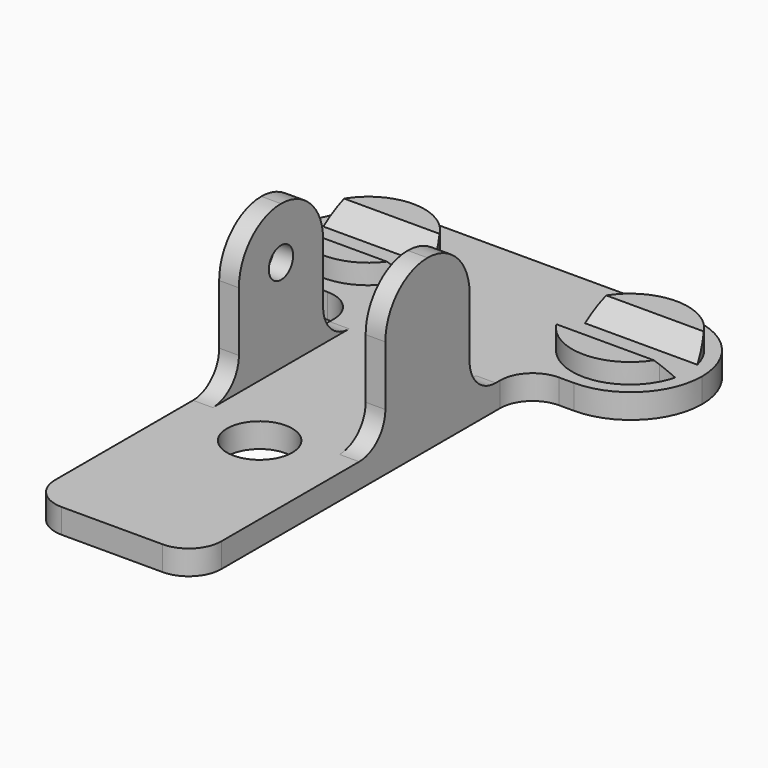
from build123d import *

# Parameters (mm, degrees)
F0_R       = 5
F1_DEPTH   = 3.75
F0_W       = 3.02
F0_H       = 16.12
F2_DEPTH   = 25.93
F3_DEPTH   = 6.79
F4_DEPTH   = 6.79
F5_SIZE2   = 3.03999
F5_SIZE    = 2.64999
F5_2_SIZE2 = 3.03999
F5_2_SIZE  = 2.64999
F6_SIZE2   = 2.64999
F6_SIZE    = 3.03999
F6_2_SIZE2 = 2.64999
F6_2_SIZE  = 3.03999
F7_R       = 2.33
F8_DEPTH   = 25
F9_R       = 8.05999
F10_R      = 5
F11_R      = 10.89999


# Not quite as in the source:
# - a fillet or chamfer is up to 0.001 mm smaller than in the source, because OpenCascade refuses the exact size


with BuildPart() as f1:
    # F0 (on Top) → F1 (new body)
    with BuildSketch(Plane.XY):
        Polygon((-30.935, 0), (-12.725, 0), (12.725, 0), (30.935, 0), (30.935, 21.8), (-30.935, 21.8), align=None)
        with BuildLine():
            ThreePointArc((-11.9316907323, 12.91), (-11.7843146524, 12.0027843216), (-11.735, 11.085))
            ThreePointArc((-11.735, 11.085), (-11.8230688054, 9.8599030561), (-12.0854641032, 8.66))
            ThreePointArc((-12.0854641032, 8.66), (-12.4738263465, 7.6050242897), (-12.9970143092, 6.61))
            ThreePointArc((-12.9970143092, 6.61), (-20.3, 2.52), (-27.6029856908, 6.61))
            ThreePointArc((-27.6029856908, 6.61), (-28.1261736535, 7.6050242897), (-28.5145358968, 8.66))
            ThreePointArc((-28.5145358968, 8.66), (-28.8593991283, 10.7753040808), (-28.6683092677, 12.91))
            ThreePointArc((-28.6683092677, 12.91), (-28.2468859573, 14.2797188579), (-27.6029856908, 15.56))
            ThreePointArc((-27.6029856908, 15.56), (-20.3, 19.65), (-12.9970143092, 15.56))
            ThreePointArc((-12.9970143092, 15.56), (-12.3531140427, 14.2797188579), (-11.9316907323, 12.91))
        make_face(mode=Mode.SUBTRACT)
        with BuildLine():
            ThreePointArc((28.6065440218, 12.91), (28.8001487986, 11.8553299132), (28.865, 10.785))
            ThreePointArc((28.865, 10.785), (28.8001487986, 9.7146700868), (28.6065440218, 8.66))
            ThreePointArc((28.6065440218, 8.66), (28.2771488358, 7.6105658536), (27.8203324738, 6.61))
            ThreePointArc((27.8203324738, 6.61), (20, 1.92), (12.1796675262, 6.61))
            ThreePointArc((12.1796675262, 6.61), (11.7228511642, 7.6105658536), (11.3934559782, 8.66))
            ThreePointArc((11.3934559782, 8.66), (11.135, 10.785), (11.3934559782, 12.91))
            ThreePointArc((11.3934559782, 12.91), (11.8536949602, 14.2815610531), (12.5308902806, 15.56))
            ThreePointArc((12.5308902806, 15.56), (20, 19.65), (27.4691097194, 15.56))
            ThreePointArc((27.4691097194, 15.56), (28.1463050398, 14.2815610531), (28.6065440218, 12.91))
        make_face(mode=Mode.SUBTRACT)
        Polygon((12.725, 0), (-12.725, 0), (-12.725, -10.84), (-9.705, -10.84), (-9.705, -26.96), (-12.725, -26.96), (-12.725, -63.35), (12.725, -63.35), (12.725, -26.96), (9.705, -26.96), (9.705, -10.84), (12.725, -10.84), align=None)
        with Locations((0, -35.12)):
            Circle(F0_R, mode=Mode.SUBTRACT)
        with BuildLine():
            ThreePointArc((-12.0854641032, 8.66), (-11.8230688054, 9.8599030561), (-11.735, 11.085))
            ThreePointArc((-11.735, 11.085), (-11.7843146524, 12.0027843216), (-11.9316907323, 12.91))
            Line((-11.9316907323, 12.91), (-28.6683092677, 12.91))
            ThreePointArc((-28.6683092677, 12.91), (-28.8593991283, 10.7753040808), (-28.5145358968, 8.66))
            Line((-28.5145358968, 8.66), (-12.0854641032, 8.66))
        make_face()
        with BuildLine():
            ThreePointArc((28.6065440218, 8.66), (28.8001487986, 9.7146700868), (28.865, 10.785))
            ThreePointArc((28.865, 10.785), (28.8001487986, 11.8553299132), (28.6065440218, 12.91))
            Line((28.6065440218, 12.91), (11.3934559782, 12.91))
            ThreePointArc((11.3934559782, 12.91), (11.135, 10.785), (11.3934559782, 8.66))
            Line((11.3934559782, 8.66), (28.6065440218, 8.66))
        make_face()
    extrude(amount=F1_DEPTH)

    # F0 (on Top) → F2 (join)
    with BuildSketch(Plane.XY):
        with Locations((-11.215, -18.9)):
            Rectangle(F0_W, F0_H)
        with Locations((11.215, -18.9)):
            Rectangle(F0_W, F0_H)
    extrude(amount=F2_DEPTH)

    # F0 (on Top) → F3 (join)
    with BuildSketch(Plane.XY):
        with BuildLine():
            Line((-27.6029856908, 15.56), (-12.9970143092, 15.56))
            ThreePointArc((-12.9970143092, 15.56), (-20.3, 19.65), (-27.6029856908, 15.56))
        make_face()
        with BuildLine():
            ThreePointArc((-27.6029856908, 6.61), (-20.3, 2.52), (-12.9970143092, 6.61))
            Line((-12.9970143092, 6.61), (-27.6029856908, 6.61))
        make_face()
        with BuildLine():
            ThreePointArc((12.1796675262, 6.61), (20, 1.92), (27.8203324738, 6.61))
            Line((27.8203324738, 6.61), (12.1796675262, 6.61))
        make_face()
        with BuildLine():
            Line((12.5308902806, 15.56), (27.4691097194, 15.56))
            ThreePointArc((27.4691097194, 15.56), (20, 19.65), (12.5308902806, 15.56))
        make_face()
    extrude(amount=F3_DEPTH)

    # F0 (on Top) → F4 (join)
    with BuildSketch(Plane.XY):
        with BuildLine():
            Line((-28.6683092677, 12.91), (-11.9316907323, 12.91))
            ThreePointArc((-11.9316907323, 12.91), (-12.3531140427, 14.2797188579), (-12.9970143092, 15.56))
            Line((-12.9970143092, 15.56), (-27.6029856908, 15.56))
            ThreePointArc((-27.6029856908, 15.56), (-28.2468859573, 14.2797188579), (-28.6683092677, 12.91))
        make_face()
        with BuildLine():
            ThreePointArc((-12.9970143092, 6.61), (-12.4738263465, 7.6050242897), (-12.0854641032, 8.66))
            Line((-12.0854641032, 8.66), (-28.5145358968, 8.66))
            ThreePointArc((-28.5145358968, 8.66), (-28.1261736535, 7.6050242897), (-27.6029856908, 6.61))
            Line((-27.6029856908, 6.61), (-12.9970143092, 6.61))
        make_face()
        with BuildLine():
            ThreePointArc((27.8203324738, 6.61), (28.2771488358, 7.6105658536), (28.6065440218, 8.66))
            Line((28.6065440218, 8.66), (11.3934559782, 8.66))
            ThreePointArc((11.3934559782, 8.66), (11.7228511642, 7.6105658536), (12.1796675262, 6.61))
            Line((12.1796675262, 6.61), (27.8203324738, 6.61))
        make_face()
        with BuildLine():
            Line((11.3934559782, 12.91), (28.6065440218, 12.91))
            ThreePointArc((28.6065440218, 12.91), (28.1463050398, 14.2815610531), (27.4691097194, 15.56))
            Line((27.4691097194, 15.56), (12.5308902806, 15.56))
            ThreePointArc((12.5308902806, 15.56), (11.8536949602, 14.2815610531), (11.3934559782, 12.91))
        make_face()
    extrude(amount=F4_DEPTH)

    # F5 (size 2.65 and 3.04 in the source; OpenCascade refuses exactly that, so slightly less here)
    f5_edges = [f1.edges().sort_by_distance(p)[0] for p in [
        (-20.3, 12.91, 6.79),
    ]]
    f5_side = f1.faces().sort_by_distance((-20.3, 15.724453, 6.79))[0]
    chamfer(f5_edges, length=F5_SIZE, length2=F5_SIZE2, reference=f5_side)

    # F5#2 (size 2.65 and 3.04 in the source; OpenCascade refuses exactly that, so slightly less here)
    f5_2_edges = [f1.edges().sort_by_distance(p)[0] for p in [
        (20, 12.91, 6.79),
    ]]
    f5_2_side = f1.faces().sort_by_distance((20, 15.719253, 6.79))[0]
    chamfer(f5_2_edges, length=F5_2_SIZE, length2=F5_2_SIZE2, reference=f5_2_side)

    # F6 (size 3.04 and 2.65 in the source; OpenCascade refuses exactly that, so slightly less here)
    f6_edges = [f1.edges().sort_by_distance(p)[0] for p in [
        (-20.3, 8.66, 6.79),
    ]]
    f6_side = f1.faces().sort_by_distance((-20.3, 8.66, 5.27))[0]
    chamfer(f6_edges, length=F6_SIZE, length2=F6_SIZE2, reference=f6_side)

    # F6#2 (size 3.04 and 2.65 in the source; OpenCascade refuses exactly that, so slightly less here)
    f6_2_edges = [f1.edges().sort_by_distance(p)[0] for p in [
        (20, 8.66, 6.79),
    ]]
    f6_2_side = f1.faces().sort_by_distance((20, 8.66, 5.27))[0]
    chamfer(f6_2_edges, length=F6_2_SIZE, length2=F6_2_SIZE2, reference=f6_2_side)

    # F7 (on face) → F8 (cut)
    with BuildSketch(Plane(origin=(-12.725, 0, 0), x_dir=(0, -1, 0), z_dir=(-1, 0, 0))):
        with Locations((18.9, 17.99)):
            Circle(F7_R)
    extrude(amount=-F8_DEPTH, mode=Mode.SUBTRACT)

    # F9 (radius 8.06 in the source; OpenCascade refuses exactly that, so slightly less here)
    f9_edges = [f1.edges().sort_by_distance(p)[0] for p in [
        (-11.215, -10.84, 25.93),
        (11.215, -10.84, 25.93),
        (11.215, -26.96, 25.93),
        (-11.215, -26.96, 25.93),
    ]]
    fillet(f9_edges, radius=F9_R)

    # F10
    f10_edges = [f1.edges().sort_by_distance(p)[0] for p in [
        (-12.725, 0, 1.875),
        (12.725, 0, 1.875),
        (12.725, -63.35, 1.875),
        (-12.725, -63.35, 1.875),
        (-11.215, -26.96, 3.75),
        (11.215, -26.96, 3.75),
        (11.215, -10.84, 3.75),
        (-11.215, -10.84, 3.75),
    ]]
    fillet(f10_edges, radius=F10_R)

    # F11 (radius 10.9 in the source; OpenCascade refuses exactly that, so slightly less here)
    f11_edges = [f1.edges().sort_by_distance(p)[0] for p in [
        (-30.935, 21.8, 1.875),
        (-30.935, 0, 1.875),
        (30.935, 21.8, 1.875),
        (30.935, 0, 1.875),
    ]]
    fillet(f11_edges, radius=F11_R)


solid = f1.part
